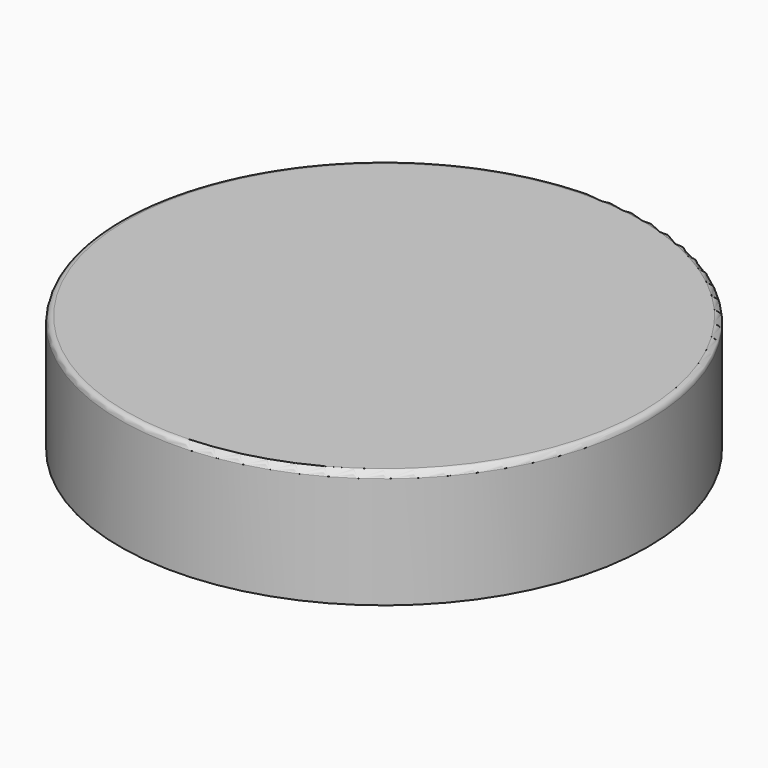
from build123d import *

# Parameters (mm, degrees)
F0_R     = 45
F1_DEPTH = 20
F2_T     = -2
F3_R     = 12
F4_DEPTH = 18
F5_T     = -2
F7_DEPTH = 18
F8_R     = 1


# Not quite as in the source:
# - a shell that OpenCascade refuses in one call is made with other operations: the cavity is built on its own and cut out


with BuildPart() as f1:
    # F0 (on Top) → F1 (new body)
    with BuildSketch(Plane.XY):
        Circle(F0_R)
    extrude(amount=F1_DEPTH)

    # F2
    f2_openings = [f1.faces().sort_by_distance(p)[0] for p in [
        (0, 0, 0),
    ]]
    offset(amount=F2_T, openings=f2_openings)

    # F3 (on Top) → F4 (join, through all)
    with BuildSketch(Plane.XY):
        Circle(F3_R)
    extrude(amount=F4_DEPTH)

    # F5: a shell. OpenCascade refuses it in one call, so the cavity is built on its own and cut out:
    # the body offset inwards by the wall thickness, plus a prism from it out through each open face.
    f5_core = offset(f1.part, amount=F5_T, kind=Kind.INTERSECTION, mode=Mode.PRIVATE)
    f5_exits = [f5_core.faces().sort_by_distance(p)[0] for p in [
        (0, 0, 2),
    ]]
    add(f5_core, mode=Mode.SUBTRACT)
    extrude(f5_exits, amount=-F5_T, mode=Mode.SUBTRACT)

    # F6 (on face) → F7 (cut, through all)
    with BuildSketch(Plane(origin=(0, 0, 0), x_dir=(1, 0, 0), z_dir=(0, 0, -1))):
        with BuildLine():
            ThreePointArc((10, 0), (9.9202969627, -1.2600429248), (9.6824583655, -2.5))
            Line((9.6824583655, -2.5), (11.7366945943, -2.5))
            ThreePointArc((11.7366945943, -2.5), (11.9339921052, -1.2569138531), (12, 0))
            ThreePointArc((12, 0), (11.9339921052, 1.2569138531), (11.7366945943, 2.5))
            Line((11.7366945943, 2.5), (9.6824583655, 2.5))
            ThreePointArc((9.6824583655, 2.5), (9.9202969627, 1.2600429248), (10, 0))
        make_face()
    extrude(amount=-F7_DEPTH, mode=Mode.SUBTRACT)

    # F8
    f8_edges = [f1.edges().sort_by_distance(p)[0] for p in [
        (-45, 0, 20),
    ]]
    fillet(f8_edges, radius=F8_R)


solid = f1.part
